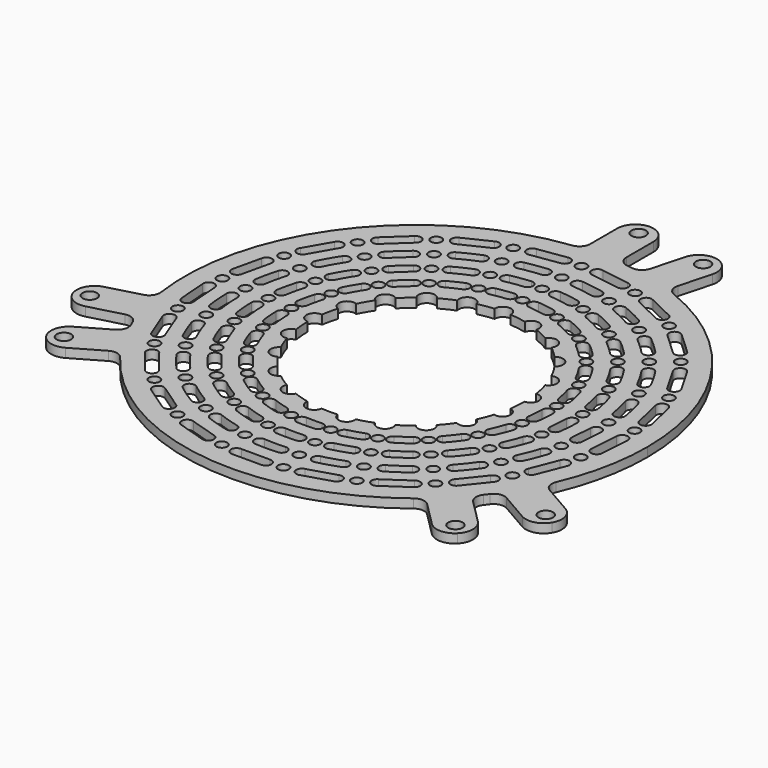
from build123d import *

# Parameters (mm, degrees)
F0_R      = 1.5
F0_R_2    = 30
F0_R_3    = 2
F1_DEPTH  = 2.5
F2_R      = 4.99999
F3_R      = 3
F5_DEPTH  = 25
F6_R      = 1.5579033755
F6_R_2    = 1.5577764336
F7_DEPTH  = 25
F8_R      = 2.25
F9_DEPTH  = 25
F11_DEPTH = 25
F12_R     = 1.5
F12_R_2   = 1.5000000369
F12_R_3   = 1.5000000493
F12_R_4   = 1.5000000692
F13_DEPTH = 25


# Not quite as in the source:
# - a fillet or chamfer is up to 0.001 mm smaller than in the source, because OpenCascade refuses the exact size


with BuildPart() as f1:
    # F0 (on Top) → F1 (new body)
    with BuildSketch(Plane.XY):
        with BuildLine():
            ThreePointArc((57.7562213692, -27.572067263), (62.4195408812, -14.1350951955), (64, 0))
            ThreePointArc((64, 0), (52.2588695026, 36.9460492923), (21.3434200529, 60.3362115188))
            ThreePointArc((21.3434200529, 60.3362115188), (16.5644188866, 61.8192528825), (11.68416179, 62.9244019699))
            ThreePointArc((11.68416179, 62.9244019699), (8.3536763021, 63.4524711279), (5, 63.8043885638))
            ThreePointArc((5, 63.8043885638), (0, 64), (-5, 63.8043885638))
            ThreePointArc((-5, 63.8043885638), (-50.7746137786, 38.9607314566), (-62.9244019699, -11.68416179))
            ThreePointArc((-62.9244019699, -11.68416179), (-61.8192528825, -16.5644188866), (-60.3362115188, -21.3434200529))
            ThreePointArc((-60.3362115188, -21.3434200529), (-59.1282900807, -24.4917396714), (-57.7562213692, -27.572067263))
            ThreePointArc((-57.7562213692, -27.572067263), (-55.4256258422, -32), (-52.7562213692, -36.2323213008))
            ThreePointArc((-52.7562213692, -36.2323213008), (-8.3536763021, -63.4524711279), (41.580981917, -48.6520497289))
            ThreePointArc((41.580981917, -48.6520497289), (45.2548339959, -45.2548339959), (48.6520497289, -41.580981917))
            ThreePointArc((48.6520497289, -41.580981917), (50.7746137786, -38.9607314566), (52.7562213692, -36.2323213008))
            ThreePointArc((52.7562213692, -36.2323213008), (55.4256258422, -32), (57.7562213692, -27.572067263))
        make_face()
        with Locations((-49.5366530965, -28.6)):
            Circle(F0_R, mode=Mode.SUBTRACT)
        with Locations((-24.8181498775, -51.535419244)):
            Circle(F0_R, mode=Mode.SUBTRACT)
        with Locations((-8.5252176253, -56.5611232601)):
            Circle(F0_R, mode=Mode.SUBTRACT)
        with Locations((-7.5117302153, -49.8370736417)):
            Circle(F0_R, mode=Mode.SUBTRACT)
        with Locations((-38.9058806005, -41.9305670687)):
            Circle(F0_R, mode=Mode.SUBTRACT)
        with Locations((-34.2807059837, -36.9458143402)):
            Circle(F0_R, mode=Mode.SUBTRACT)
        with Locations((-29.6555313668, -31.9610616118)):
            Circle(F0_R, mode=Mode.SUBTRACT)
        with Locations((-21.8677404515, -45.4088309423)):
            Circle(F0_R, mode=Mode.SUBTRACT)
        with Locations((-18.9173310255, -39.2822426405)):
            Circle(F0_R, mode=Mode.SUBTRACT)
        with Locations((-6.4982428053, -43.1130240234)):
            Circle(F0_R, mode=Mode.SUBTRACT)
        with Locations((-15.9669215995, -33.1556543388)):
            Circle(F0_R, mode=Mode.SUBTRACT)
        with Locations((-5.4847553953, -36.3889744051)):
            Circle(F0_R, mode=Mode.SUBTRACT)
        with Locations((-43.6476803507, -25.2)):
            Circle(F0_R, mode=Mode.SUBTRACT)
        with Locations((-55.7658765768, -12.7281974223)):
            Circle(F0_R, mode=Mode.SUBTRACT)
        with Locations((-49.136366774, -11.2150550714)):
            Circle(F0_R, mode=Mode.SUBTRACT)
        with Locations((-42.5068569711, -9.7019127205)):
            Circle(F0_R, mode=Mode.SUBTRACT)
        with Locations((-57.0400571988, 4.2745613531)):
            Circle(F0_R, mode=Mode.SUBTRACT)
        with Locations((-50.2590713779, 3.7663967168)):
            Circle(F0_R, mode=Mode.SUBTRACT)
        with Locations((-43.4780855571, 3.2582320804)):
            Circle(F0_R, mode=Mode.SUBTRACT)
        with Locations((-37.758707605, -21.8)):
            Circle(F0_R, mode=Mode.SUBTRACT)
        with Locations((-25.03035675, -26.9763088833)):
            Circle(F0_R, mode=Mode.SUBTRACT)
        with Locations((-31.8697348593, -18.4)):
            Circle(F0_R, mode=Mode.SUBTRACT)
        with Locations((-35.8773471683, -8.1887703696)):
            Circle(F0_R, mode=Mode.SUBTRACT)
        with Locations((-36.6970997363, 2.750067444)):
            Circle(F0_R, mode=Mode.SUBTRACT)
        with Locations((8.5252176253, -56.5611232601)):
            Circle(F0_R, mode=Mode.SUBTRACT)
        with Locations((7.5117302153, -49.8370736417)):
            Circle(F0_R, mode=Mode.SUBTRACT)
        with Locations((24.8181498775, -51.535419244)):
            Circle(F0_R, mode=Mode.SUBTRACT)
        with Locations((6.4982428053, -43.1130240234)):
            Circle(F0_R, mode=Mode.SUBTRACT)
        with Locations((5.4847553953, -36.3889744051)):
            Circle(F0_R, mode=Mode.SUBTRACT)
        with Locations((21.8677404515, -45.4088309423)):
            Circle(F0_R, mode=Mode.SUBTRACT)
        with Locations((18.9173310255, -39.2822426405)):
            Circle(F0_R, mode=Mode.SUBTRACT)
        with Locations((34.2807059837, -36.9458143402)):
            Circle(F0_R, mode=Mode.SUBTRACT)
        with Locations((15.9669215995, -33.1556543388)):
            Circle(F0_R, mode=Mode.SUBTRACT)
        with Locations((29.6555313668, -31.9610616118)):
            Circle(F0_R, mode=Mode.SUBTRACT)
        with Locations((38.9058806005, -41.9305670687)):
            Circle(F0_R, mode=Mode.SUBTRACT)
        with Locations((49.5366530965, -28.6)):
            Circle(F0_R, mode=Mode.SUBTRACT)
        with Locations((25.03035675, -26.9763088833)):
            Circle(F0_R, mode=Mode.SUBTRACT)
        with Locations((31.8697348593, -18.4)):
            Circle(F0_R, mode=Mode.SUBTRACT)
        Circle(F0_R_2, mode=Mode.SUBTRACT)
        with Locations((43.6476803507, -25.2)):
            Circle(F0_R, mode=Mode.SUBTRACT)
        with Locations((37.758707605, -21.8)):
            Circle(F0_R, mode=Mode.SUBTRACT)
        with Locations((42.5068569711, -9.7019127205)):
            Circle(F0_R, mode=Mode.SUBTRACT)
        with Locations((49.136366774, -11.2150550714)):
            Circle(F0_R, mode=Mode.SUBTRACT)
        with Locations((55.7658765768, -12.7281974223)):
            Circle(F0_R, mode=Mode.SUBTRACT)
        with Locations((35.8773471683, -8.1887703696)):
            Circle(F0_R, mode=Mode.SUBTRACT)
        with Locations((36.6970997363, 2.750067444)):
            Circle(F0_R, mode=Mode.SUBTRACT)
        with Locations((43.4780855571, 3.2582320804)):
            Circle(F0_R, mode=Mode.SUBTRACT)
        with Locations((50.2590713779, 3.7663967168)):
            Circle(F0_R, mode=Mode.SUBTRACT)
        with Locations((57.0400571988, 4.2745613531)):
            Circle(F0_R, mode=Mode.SUBTRACT)
        with Locations((-53.2459784224, 20.8975065938)):
            Circle(F0_R, mode=Mode.SUBTRACT)
        with Locations((-46.9160369317, 18.4131876281)):
            Circle(F0_R, mode=Mode.SUBTRACT)
        with Locations((-44.7207607972, 35.6636166663)):
            Circle(F0_R, mode=Mode.SUBTRACT)
        with Locations((-40.5860954409, 15.9288686624)):
            Circle(F0_R, mode=Mode.SUBTRACT)
        with Locations((-34.2561539501, 13.4445496967)):
            Circle(F0_R, mode=Mode.SUBTRACT)
        with Locations((-28.7713985548, 22.9444247084)):
            Circle(F0_R, mode=Mode.SUBTRACT)
        with Locations((-34.0878526356, 27.184155361)):
            Circle(F0_R, mode=Mode.SUBTRACT)
        with Locations((-39.4043067164, 31.4238860137)):
            Circle(F0_R, mode=Mode.SUBTRACT)
        with Locations((-24.5607545316, 36.0240105602)):
            Circle(F0_R, mode=Mode.SUBTRACT)
        with Locations((-28.3913309264, 41.6424342255)):
            Circle(F0_R, mode=Mode.SUBTRACT)
        with Locations((-20.7301781367, 30.4055868948)):
            Circle(F0_R, mode=Mode.SUBTRACT)
        with Locations((-10.8469904183, 35.1650792529)):
            Circle(F0_R, mode=Mode.SUBTRACT)
        with Locations((-12.8513256043, 41.6629743323)):
            Circle(F0_R, mode=Mode.SUBTRACT)
        with Locations((-32.2219073212, 47.2608578909)):
            Circle(F0_R, mode=Mode.SUBTRACT)
        with Locations((-14.8556607903, 48.1608694116)):
            Circle(F0_R, mode=Mode.SUBTRACT)
        with Locations((-16.8599959763, 54.658764491)):
            Circle(F0_R, mode=Mode.SUBTRACT)
        with Locations((34.2561539501, 13.4445496967)):
            Circle(F0_R, mode=Mode.SUBTRACT)
        with Locations((28.7713985548, 22.9444247084)):
            Circle(F0_R, mode=Mode.SUBTRACT)
        with Locations((10.8469904183, 35.1650792529)):
            Circle(F0_R, mode=Mode.SUBTRACT)
        with Locations((0, 36.8)):
            Circle(F0_R, mode=Mode.SUBTRACT)
        with Locations((0, 43.6)):
            Circle(F0_R, mode=Mode.SUBTRACT)
        with Locations((12.8513256043, 41.6629743323)):
            Circle(F0_R, mode=Mode.SUBTRACT)
        with Locations((20.7301781367, 30.4055868948)):
            Circle(F0_R, mode=Mode.SUBTRACT)
        with Locations((34.0878526356, 27.184155361)):
            Circle(F0_R, mode=Mode.SUBTRACT)
        with Locations((24.5607545316, 36.0240105602)):
            Circle(F0_R, mode=Mode.SUBTRACT)
        with Locations((28.3913309264, 41.6424342255)):
            Circle(F0_R, mode=Mode.SUBTRACT)
        with Locations((40.5860954409, 15.9288686624)):
            Circle(F0_R, mode=Mode.SUBTRACT)
        with Locations((46.9160369317, 18.4131876281)):
            Circle(F0_R, mode=Mode.SUBTRACT)
        with Locations((53.2459784224, 20.8975065938)):
            Circle(F0_R, mode=Mode.SUBTRACT)
        with Locations((39.4043067164, 31.4238860137)):
            Circle(F0_R, mode=Mode.SUBTRACT)
        with Locations((44.7207607972, 35.6636166663)):
            Circle(F0_R, mode=Mode.SUBTRACT)
        with Locations((0, 50.4)):
            Circle(F0_R, mode=Mode.SUBTRACT)
        with Locations((14.8556607903, 48.1608694116)):
            Circle(F0_R, mode=Mode.SUBTRACT)
        with Locations((0, 57.2)):
            Circle(F0_R, mode=Mode.SUBTRACT)
        with Locations((32.2219073212, 47.2608578909)):
            Circle(F0_R, mode=Mode.SUBTRACT)
        with Locations((16.8599959763, 54.658764491)):
            Circle(F0_R, mode=Mode.SUBTRACT)
        with BuildLine():
            ThreePointArc((-5, 63.8043885638), (0, 64), (5, 63.8043885638))
            Line((5, 63.8043885638), (5, 80.8455317256))
            Line((5, 80.8455317256), (-5, 80.8455317256))
            Line((-5, 80.8455317256), (-5, 63.8043885638))
        make_face()
        with Locations((0, 77)):
            Circle(F0_R_3, mode=Mode.SUBTRACT)
        with BuildLine():
            ThreePointArc((11.68416179, 62.9244019699), (16.5644188866, 61.8192528825), (21.3434200529, 60.3362115188))
            Line((21.3434200529, 60.3362115188), (25.7539924535, 76.7966918083))
            Line((25.7539924535, 76.7966918083), (16.0947341906, 79.3848822594))
            Line((16.0947341906, 79.3848822594), (11.68416179, 62.9244019699))
        make_face()
        with Locations((19.9290664729, 74.3762886243)):
            Circle(F0_R_3, mode=Mode.SUBTRACT)
        with BuildLine():
            Line((72.5142842569, -36.0926388439), (57.7562213692, -27.572067263))
            ThreePointArc((57.7562213692, -27.572067263), (55.4256258422, -32), (52.7562213692, -36.2323213008))
            Line((52.7562213692, -36.2323213008), (67.5142842569, -44.7528928817))
            Line((67.5142842569, -44.7528928817), (72.5142842569, -36.0926388439))
        make_face()
        with Locations((66.6839560914, -38.5)):
            Circle(F0_R_3, mode=Mode.SUBTRACT)
        with BuildLine():
            Line((60.7019576178, -53.6308898059), (48.6520497289, -41.580981917))
            ThreePointArc((48.6520497289, -41.580981917), (45.2548339959, -45.2548339959), (41.580981917, -48.6520497289))
            Line((41.580981917, -48.6520497289), (53.6308898059, -60.7019576178))
            Line((53.6308898059, -60.7019576178), (60.7019576178, -53.6308898059))
        make_face()
        with Locations((54.4472221514, -54.4472221514)):
            Circle(F0_R_3, mode=Mode.SUBTRACT)
        with BuildLine():
            Line((-67.5142842569, -44.7528928817), (-52.7562213692, -36.2323213008))
            ThreePointArc((-52.7562213692, -36.2323213008), (-55.4256258422, -32), (-57.7562213692, -27.572067263))
            Line((-57.7562213692, -27.572067263), (-72.5142842569, -36.0926388439))
            Line((-72.5142842569, -36.0926388439), (-67.5142842569, -44.7528928817))
        make_face()
        with Locations((-66.6839560914, -38.5)):
            Circle(F0_R_3, mode=Mode.SUBTRACT)
        with BuildLine():
            ThreePointArc((-60.3362115188, -21.3434200529), (-61.8192528825, -16.5644188866), (-62.9244019699, -11.68416179))
            Line((-62.9244019699, -11.68416179), (-79.3848822594, -16.0947341906))
            Line((-79.3848822594, -16.0947341906), (-76.7966918083, -25.7539924535))
            Line((-76.7966918083, -25.7539924535), (-60.3362115188, -21.3434200529))
        make_face()
        with Locations((-74.3762886243, -19.9290664729)):
            Circle(F0_R_3, mode=Mode.SUBTRACT)
    extrude(amount=F1_DEPTH)

    # F2 (radius 5 in the source; OpenCascade refuses exactly that, so slightly less here)
    f2_edges = [f1.edges().sort_by_distance(p)[0] for p in [
        (-5, 80.845532, 1.25),
        (5, 80.845532, 1.25),
        (16.094734, 79.384882, 1.25),
        (25.753992, 76.796692, 1.25),
        (-67.514284, -44.752893, 1.25),
        (-72.514284, -36.092639, 1.25),
        (-76.796692, -25.753992, 1.25),
        (-79.384882, -16.094734, 1.25),
        (60.701958, -53.63089, 1.25),
        (53.63089, -60.701958, 1.25),
        (67.514284, -44.752893, 1.25),
        (72.514284, -36.092639, 1.25),
    ]]
    fillet(f2_edges, radius=F2_R)

    # F3
    f3_edges = [f1.edges().sort_by_distance(p)[0] for p in [
        (5, 63.804389, 1.25),
        (-5, 63.804389, 1.25),
        (-57.756221, -27.572067, 1.25),
        (-62.924402, -11.684162, 1.25),
        (-52.756221, -36.232321, 1.25),
        (-60.336212, -21.34342, 1.25),
        (21.34342, 60.336212, 1.25),
        (11.684162, 62.924402, 1.25),
        (57.756221, -27.572067, 1.25),
        (48.65205, -41.580982, 1.25),
        (52.756221, -36.232321, 1.25),
        (41.580982, -48.65205, 1.25),
    ]]
    fillet(f3_edges, radius=F3_R)

    # F4 (on face) → F5 (cut)
    with BuildSketch(Plane.XY.offset(2.5)):
        Polygon((-36.8119077732, 45.824213326), (-42.9265368297, 40.1533001964), (-40.65668766, 38.01918342), (-34.8915175, 43.3705725804), align=None)
        Polygon((-48.6833819883, 32.9378718048), (-52.8548242436, 25.7165828801), (-50.0567761412, 24.3463287121), (-46.1250859609, 31.159284403), align=None)
        Polygon((-56.2291240703, 17.1248558283), (-58.0867285739, 8.9948343196), (-55.0091003916, 8.5101958561), (-53.2602381175, 16.1793570661), align=None)
        Polygon((-58.7786617212, -0.2097787398), (-58.1573721609, -8.5261447434), (-55.0736246688, -8.0821052481), (-55.6629843887, -0.238177148), align=None)
        Polygon((-56.1054573322, -17.5257735462), (-53.0604780121, -25.2895384295), (-50.2446157076, -23.9562758333), (-53.1198302239, -16.6345482773), align=None)
        Polygon((-48.4470368446, -33.2845264625), (-43.2489275398, -39.8058456449), (-40.9511521459, -37.7018261803), (-45.8567460312, -31.5528667926), align=None)
        Polygon((-36.4838845269, -46.0858031359), (-29.5945200608, -50.7852287897), (-28.0189990048, -48.0974038195), (-34.5190887147, -43.667574626), align=None)
        Polygon((-21.2789789622, -54.7921539564), (-13.310509601, -57.2521214892), (-12.5972348428, -54.2193160573), (-20.1142588813, -51.9022268218), align=None)
        Polygon((-4.1833427354, -58.6299814464), (4.1561980491, -58.6319119476), (3.943848917, -55.5236041259), (-3.9221888763, -55.5251383954), align=None)
        Polygon((13.2840018517, -57.2582777916), (21.2536092633, -54.8019997275), (20.1345043932, -51.8943763065), (12.6183848226, -54.2143977544), align=None)
        Polygon((29.5710045784, -50.7989248811), (36.4625440246, -46.102689337), (34.5361207953, -43.6541054177), (28.0377596551, -48.086469957), align=None)
        Polygon((43.2304937781, -39.8258645675), (48.431621736, -33.3069526807), (45.8690513055, -31.5349756895), (40.9658565006, -37.68584828), align=None)
        Polygon((53.0487638918, -25.3141014142), (56.0973373175, -17.5517471134), (53.1263153142, -16.6138249824), (50.2539572203, -23.9366736016), align=None)
        Polygon((58.1534185329, -8.5530692611), (58.7785582993, -0.2369917906), (55.6630730662, -0.2164630171), (55.0767733051, -8.0606204294), align=None)
        Polygon((58.0908867354, 8.9679406303), (56.2370464307, 17.0988212928), (53.2539225029, 16.2001326373), (55.0057763813, 8.5316542414), align=None)
        Polygon((52.8667247237, 25.6921096416), (48.6986261945, 32.9153290674), (46.1129272242, 31.1772754137), (50.0472748372, 24.3658539924), align=None)
        Polygon((42.9451222186, 40.1334219633), (36.8331193106, 45.8071654079), (34.8745959984, 43.3841804504), (40.6418532949, 38.0350406883), align=None)
        Polygon((29.2076571427, 51.0087036209), (21.6948281364, 54.6288340804), (20.5375038735, 51.7362106658), (27.6252247336, 48.324647105), align=None)
        Polygon((12.8749635541, 57.3516381138), (4.6288562761, 58.5964911102), (4.3755644021, 55.4912515228), (12.1539737234, 54.3203965573), align=None)
        Polygon((-4.6017270472, 58.5986278767), (-12.8484097777, 57.3575927584), (-12.1751631683, 54.3156511627), (-4.397211189, 55.4895403942), align=None)
        Polygon((-21.669534006, 54.638872397), (-29.1840382385, 51.0222205803), (-27.6440740613, 48.3138668365), (-20.5576845904, 51.7281950554), align=None)
    extrude(amount=-F5_DEPTH, mode=Mode.SUBTRACT)

    # F6 (on face) → F7 (cut)
    with BuildSketch(Plane.XY.offset(2.5)):
        with Locations((-57.2208230549, -0.2239779439)):
            Circle(F6_R)
        with Locations((-56.6154984149, -8.3041249957)):
            Circle(F6_R_2)
        with Locations((-54.6126437781, -17.0801609118)):
            Circle(F6_R)
        with Locations((-51.6525468599, -24.6229071314)):
            Circle(F6_R_2)
        with Locations((-47.1518914379, -32.4186966276)):
            Circle(F6_R)
        with Locations((-42.1000398428, -38.7538359126)):
            Circle(F6_R_2)
        with Locations((-35.5014866208, -44.8766888809)):
            Circle(F6_R)
        with Locations((-28.8067595328, -49.4413163046)):
            Circle(F6_R_2)
        with Locations((-20.6966189217, -53.3471903891)):
            Circle(F6_R)
        with Locations((-12.9538722219, -55.7357187732)):
            Circle(F6_R_2)
        with Locations((-4.0527658059, -57.0775599209)):
            Circle(F6_R)
        with Locations((4.050023483, -57.0777580367)):
            Circle(F6_R_2)
        with Locations((12.9511933371, -55.736337773)):
            Circle(F6_R)
        with Locations((20.6940568283, -53.348188017)):
            Circle(F6_R_2)
        with Locations((28.8043821168, -49.4426974191)):
            Circle(F6_R)
        with Locations((35.49933241, -44.8783973774)):
            Circle(F6_R_2)
        with Locations((42.0981751393, -38.7558564238)):
            Circle(F6_R)
        with Locations((47.1503365208, -32.4209641851)):
            Circle(F6_R_2)
        with Locations((51.651360556, -24.6253875079)):
            Circle(F6_R)
        with Locations((54.6118263158, -17.0827860479)):
            Circle(F6_R_2)
        with Locations((56.615095919, -8.3068448453)):
            Circle(F6_R)
        with Locations((57.2208156827, -0.2267274038)):
            Circle(F6_R_2)
        with Locations((56.5483315583, 8.7497974359)):
            Circle(F6_R)
        with Locations((54.7454844668, 16.6494769651)):
            Circle(F6_R_2)
        with Locations((51.4569997805, 25.028981817)):
            Circle(F6_R)
        with Locations((47.4057767094, 32.0463022406)):
            Circle(F6_R_2)
        with Locations((41.7934877568, 39.0842313258)):
            Circle(F6_R)
        with Locations((35.8538576545, 44.5956729292)):
            Circle(F6_R_2)
        with Locations((28.4164409382, 49.666675363)):
            Circle(F6_R)
        with Locations((21.1161660049, 53.1825223731)):
            Circle(F6_R_2)
        with Locations((12.5144686387, 55.8360173355)):
            Circle(F6_R)
        with Locations((4.5022103391, 57.0438713165)):
            Circle(F6_R_2)
        with Locations((-4.4994691181, 57.0440841355)):
            Circle(F6_R)
        with Locations((-12.511786473, 55.8366219606)):
            Circle(F6_R_2)
        with Locations((-21.1136092982, 53.1835337262)):
            Circle(F6_R)
        with Locations((-28.4140561499, 49.6680437084)):
            Circle(F6_R_2)
        with Locations((-35.8517126366, 44.5973929532)):
            Circle(F6_R)
        with Locations((-41.7916122449, 39.0862418082)):
            Circle(F6_R_2)
        with Locations((-47.4042339746, 32.0485781039)):
            Circle(F6_R)
        with Locations((-51.4558001924, 25.0314557961)):
            Circle(F6_R_2)
        with Locations((-54.7446810939, 16.6521064472)):
            Circle(F6_R)
        with Locations((-56.5479144828, 8.7525150879)):
            Circle(F6_R_2)
    extrude(amount=-F7_DEPTH, mode=Mode.SUBTRACT)

    # F8 (on face) → F9 (cut)
    with BuildSketch(Plane.XY.offset(2.5)):
        with Locations((16.8996017419, 24.7871632295)):
            Circle(F8_R)
        with Locations((8.8426552323, 28.6671841736)):
            Circle(F8_R)
        with Locations((0, 30)):
            Circle(F8_R)
        with Locations((-8.8426552323, 28.6671841736)):
            Circle(F8_R)
        with Locations((-16.8996017419, 24.7871632295)):
            Circle(F8_R)
        with Locations((-23.454944474, 18.7046940558)):
            Circle(F8_R)
        with Locations((-27.9262124593, 10.960230731)):
            Circle(F8_R)
        with Locations((-29.9161139154, 2.2419028076)):
            Circle(F8_R)
        with Locations((-29.2478373655, -6.6756280187)):
            Circle(F8_R)
        with Locations((-25.9807621135, -15)):
            Circle(F8_R)
        with Locations((-20.4051821331, -21.9915561549)):
            Circle(F8_R)
        with Locations((-13.0165121735, -27.0290660371)):
            Circle(F8_R)
        with Locations((-4.4712679853, -29.6649247868)):
            Circle(F8_R)
        with Locations((4.4712679853, -29.6649247868)):
            Circle(F8_R)
        with Locations((13.0165121735, -27.0290660371)):
            Circle(F8_R)
        with Locations((20.4051821331, -21.9915561549)):
            Circle(F8_R)
        with Locations((25.9807621135, -15)):
            Circle(F8_R)
        with Locations((29.2478373655, -6.6756280187)):
            Circle(F8_R)
        with Locations((29.9161139154, 2.2419028076)):
            Circle(F8_R)
        with Locations((27.9262124593, 10.960230731)):
            Circle(F8_R)
        with Locations((23.454944474, 18.7046940558)):
            Circle(F8_R)
    extrude(amount=-F9_DEPTH, mode=Mode.SUBTRACT)

    # F10 (on face) → F11 (cut)
    with BuildSketch(Plane.XY.offset(2.5)):
        with BuildLine():
            Line((41.7169760554, -5.6660311324), (44.6896821876, -6.06978632))
            ThreePointArc((44.6896821876, -6.06978632), (44.97384885, -3.3708929995), (45.0951734833, -0.6597942959))
            Line((45.0951734833, -0.6597942959), (42.0954836602, -0.6166485343))
            Line((42.0954836602, -0.6166485343), (41.7169760554, -5.6660311324))
        make_face()
        with BuildLine():
            Line((34.9788421557, -4.7508527072), (37.9515482879, -5.1546078948))
            ThreePointArc((37.9515482879, -5.1546078948), (38.1928064688, -2.8634828512), (38.2958765288, -0.5619972359))
            Line((38.2958765288, -0.5619972359), (35.2961866658, -0.5188514737))
            ThreePointArc((35.2961866658, -0.5188514737), (35.2011701166, -2.6396254323), (34.9788421557, -4.7508527072))
        make_face()
        Polygon((51.8944703734, -0.7575913551), (48.8947805752, -0.7144455938), (48.4551099551, -6.5812095576), (51.4278160873, -6.9849647451), align=None)
        with BuildLine():
            Line((49.8122486315, 14.5722299691), (46.9331091981, 13.7292847956))
            ThreePointArc((46.9331091981, 13.7292847956), (47.6740070724, 10.881132738), (48.2422309454, 7.9935695035))
            Line((48.2422309454, 7.9935695035), (51.2018770157, 8.4839725405))
            ThreePointArc((51.2018770157, 8.4839725405), (50.5987165321, 11.5490209673), (49.8122486315, 14.5722299691))
        make_face()
        with BuildLine():
            Line((34.8251687602, 5.770409069), (37.7848148305, 6.260812106))
            ThreePointArc((37.7848148305, 6.260812106), (37.3400336254, 8.5212609895), (36.7601497779, 10.7508784899))
            Line((36.7601497779, 10.7508784899), (33.8810102824, 9.9079332983))
            ThreePointArc((33.8810102824, 9.9079332983), (34.4153241499, 7.8533727566), (34.8251687602, 5.770409069))
        make_face()
        with BuildLine():
            Line((43.2861992356, 12.6615542385), (40.4070597784, 11.8186090581))
            ThreePointArc((40.4070597784, 11.8186090581), (41.0446656208, 9.3672527495), (41.5336998528, 6.8819892863))
            Line((41.5336998528, 6.8819892863), (44.4933459231, 7.3723923233))
            ThreePointArc((44.4933459231, 7.3723923233), (43.9693750866, 10.0351409802), (43.2861992356, 12.6615542385))
        make_face()
        with BuildLine():
            Line((43.3039900013, 28.6072447113), (40.8012251063, 26.9531079809))
            ThreePointArc((40.8012251063, 26.9531079809), (42.3487145232, 24.4498748101), (43.7428180087, 21.858084835))
            Line((43.7428180087, 21.858084835), (46.4264264755, 23.1990716347))
            ThreePointArc((46.4264264755, 23.1990716347), (44.9466238363, 25.9501638862), (43.3039900013, 28.6072447113))
        make_face()
        with BuildLine():
            Line((31.5771262926, 15.7789446764), (34.2607347594, 17.1199314761))
            ThreePointArc((34.2607347594, 17.1199314761), (33.1694349305, 19.1488533963), (31.9581224, 21.1084914824))
            Line((31.9581224, 21.1084914824), (29.4553574511, 19.4543547164))
            ThreePointArc((29.4553574511, 19.4543547164), (30.5715256034, 17.6485643121), (31.5771262926, 15.7789446764))
        make_face()
        with BuildLine():
            Line((37.6310562275, 24.8578681146), (35.1282913118, 23.2037313705))
            ThreePointArc((35.1282913118, 23.2037313705), (36.4601200719, 21.0492195661), (37.6599721507, 18.8185147557))
            Line((37.6599721507, 18.8185147557), (40.3435806175, 20.1595015554))
            ThreePointArc((40.3435806175, 20.1595015554), (39.0580293903, 22.5495086453), (37.6310562275, 24.8578681146))
        make_face()
        with BuildLine():
            Line((25.52331758, 24.3854518045), (27.6924380542, 26.4578698049))
            ThreePointArc((27.6924380542, 26.4578698049), (26.0515863802, 28.0749861455), (24.316475601, 29.5905223737))
            Line((24.316475601, 29.5905223737), (22.4124668475, 27.2721713439))
            ThreePointArc((22.4124668475, 27.2721713439), (24.0113128461, 25.8756034791), (25.52331758, 24.3854518045))
        make_face()
        with BuildLine():
            Line((32.9479818229, 40.1003802201), (31.0439731105, 37.7820292403))
            ThreePointArc((31.0439731105, 37.7820292403), (33.2605528444, 35.8461382088), (35.3566637298, 33.7804134063))
            Line((35.3566637298, 33.7804134063), (37.525784204, 35.8528314067))
            ThreePointArc((37.525784204, 35.8528314067), (35.3008263676, 38.0455208634), (32.9479818229, 40.1003802201))
        make_face()
        with BuildLine():
            Line((28.6322287324, 34.8454513217), (26.7282200042, 32.5271003228))
            ThreePointArc((26.7282200042, 32.5271003228), (28.635932852, 30.8608708512), (30.4399906549, 29.0829326054))
            Line((30.4399906549, 29.0829326054), (32.6091111291, 31.1553506058))
            ThreePointArc((32.6091111291, 31.1553506058), (30.6762063794, 33.0602535104), (28.6322287324, 34.8454513217))
        make_face()
        with BuildLine():
            Line((17.2016500931, 30.8252045261), (18.6635467016, 33.4449102932))
            ThreePointArc((18.6635467016, 33.4449102931), (16.6189400546, 34.5065331707), (14.5142032337, 35.4433054961))
            Line((14.5142032337, 35.4433054961), (13.378130209, 32.6667358656))
            ThreePointArc((13.378130209, 32.6667358656), (15.3175895705, 31.8034817237), (17.2016500931, 30.8252045261))
        make_face()
        with BuildLine():
            Line((19.6644008698, 48.0304209687), (18.5283278696, 45.253851398))
            ThreePointArc((18.5283278696, 45.253851398), (21.2170450839, 44.0573149194), (23.8289147182, 42.7012040035))
            Line((23.8289147182, 42.7012040035), (25.2908113267, 45.3209097706))
            ThreePointArc((25.2908113267, 45.3209097706), (22.518395561, 46.7603663518), (19.6644008698, 48.0304209687))
        make_face()
        with BuildLine():
            Line((17.089302064, 41.7368632622), (15.9532290543, 38.9602936686))
            ThreePointArc((15.9532290543, 38.9602936686), (18.2673173315, 37.9303983305), (20.5152824057, 36.7632042648))
            Line((20.5152824057, 36.7632042648), (21.9771790142, 39.3829100319))
            ThreePointArc((21.9771790142, 39.3829100319), (19.5686678113, 40.6334497685), (17.089302064, 41.7368632622))
        make_face()
        with BuildLine():
            Line((7.3515405073, 34.5260025513), (7.976317321, 37.4602237313))
            ThreePointArc((7.976317321, 37.4602237312), (5.7096279742, 37.8720232942), (3.4222802146, 38.1467953848))
            Line((3.4222802146, 38.1467953848), (3.1550879925, 35.15871755))
            ThreePointArc((3.1550879925, 35.15871755), (5.2628312414, 34.9054810499), (7.3515405073, 34.5260025513))
        make_face()
        with BuildLine():
            Line((4.6335516036, 51.6927480362), (4.3663593873, 48.7046702658))
            ThreePointArc((4.3663593873, 48.7046702658), (7.2883097581, 48.3538058571), (10.1838620625, 47.8278052339))
            Line((10.1838620625, 47.8278052339), (10.8086388762, 50.7620264139))
            ThreePointArc((10.8086388762, 50.7620264139), (7.7351064885, 51.3203480854), (4.6335516036, 51.6927480362))
        make_face()
        with BuildLine():
            Line((4.027915912, 44.9197717426), (3.7607236934, 41.9316939474))
            ThreePointArc((3.7607236934, 41.9316939474), (6.2755705013, 41.6296434633), (8.7677012849, 41.1769038926))
            Line((8.7677012849, 41.1769038926), (9.3924780986, 44.1111250726))
            ThreePointArc((9.3924780986, 44.1111250726), (6.7223672325, 44.5961856978), (4.027915912, 44.9197717426))
        make_face()
        with BuildLine():
            Line((-3.1517857143, 35.1590137349), (-3.4196428571, 38.1470318993))
            ThreePointArc((-3.4196428571, 38.1470318993), (-5.7070096081, 37.8724179494), (-7.97372742, 37.4607750992))
            Line((-7.97372742, 37.4607750992), (-7.348297638, 34.5266928886))
            ThreePointArc((-7.348297638, 34.5266928886), (-5.259552739, 34.9059752046), (-3.1517857143, 35.1590137349))
        make_face()
        with BuildLine():
            Line((-10.8090090566, 50.7619475908), (-10.1835792881, 47.8278654435))
            ThreePointArc((-10.1835792881, 47.8278654435), (-7.2880238738, 48.3538489473), (-4.3660714286, 48.7046960804))
            Line((-4.3660714286, 48.7046960804), (-4.6339285714, 51.6927142448))
            ThreePointArc((-4.6339285714, 51.6927142448), (-7.7354807405, 51.320291676), (-10.8090090566, 50.7619475908))
        make_face()
        with BuildLine():
            Line((-9.391368245, 44.1113613765), (-8.7659384713, 41.1772792049))
            ThreePointArc((-8.7659384713, 41.1772792049), (-6.2737883079, 41.6299120858), (-3.7589285714, 41.9318549076))
            Line((-3.7589285714, 41.9318549076), (-4.0267857143, 44.9198730721))
            ThreePointArc((-4.0267857143, 44.9198730721), (-6.7212451755, 44.5963548207), (-9.391368245, 44.1113613765))
        make_face()
        with BuildLine():
            Line((-13.3750619438, 32.6679922554), (-14.5117527605, 35.4443088777))
            ThreePointArc((-14.5117527605, 35.4443088777), (-16.6165543419, 34.5076820694), (-18.6612343813, 33.446200552))
            Line((-18.6612343813, 33.446200552), (-17.1987547759, 30.8268200461))
            ThreePointArc((-17.1987547759, 30.8268200461), (-15.3146023774, 31.8049202801), (-13.3750619438, 32.6679922554))
        make_face()
        with BuildLine():
            Line((-25.2911418275, 45.3207253369), (-23.8286622537, 42.7013448875))
            ThreePointArc((-23.8286622537, 42.7013448875), (-21.2167846016, 44.0574403611), (-18.5280603131, 45.2539609431))
            Line((-18.5280603131, 45.2539609431), (-19.6647511298, 48.0302775653))
            ThreePointArc((-19.6647511298, 48.0302775653), (-22.5187365591, 46.7602021358), (-25.2911418275, 45.3207253369))
        make_face()
        with BuildLine():
            Line((-21.9761881201, 39.3834629726), (-20.5137085342, 36.7640825015))
            ThreePointArc((-20.5137085342, 36.7640825015), (-18.2656934938, 37.9311803295), (-15.9515611284, 38.9609765992))
            Line((-15.9515611284, 38.9609765992), (-17.0882519452, 41.7372932215))
            ThreePointArc((-17.0882519452, 41.7372932215), (-19.567645454, 40.6339421099), (-21.9761881201, 39.3834629726))
        make_face()
        with BuildLine():
            Line((-22.4099052241, 27.2742763029), (-24.3144297474, 29.5922034675))
            ThreePointArc((-24.3144297474, 29.5922034675), (-26.0496453019, 28.0767872031), (-27.6906087742, 26.4597843096))
            Line((-27.6906087742, 26.4597843096), (-25.5210270765, 24.3878489613))
            ThreePointArc((-25.5210270765, 24.3878489613), (-24.0088823876, 25.877858615), (-22.4099052241, 27.2742763029))
        make_face()
        with BuildLine():
            Line((-37.5260456588, 35.85255775), (-35.3564640078, 33.7806224464))
            ThreePointArc((-35.3564640078, 33.7806224464), (-33.2603409093, 35.8463348559), (-31.0437497297, 37.7822127822))
            Line((-31.0437497297, 37.7822127822), (-32.948274253, 40.1001399468))
            ThreePointArc((-32.948274253, 40.1001399468), (-35.3011038126, 38.0452634321), (-37.5260456588, 35.85255775))
        make_face()
        with BuildLine():
            Line((-32.6083272398, 31.156171052), (-30.4387455709, 29.0842357313))
            ThreePointArc((-30.4387455709, 29.0842357313), (-28.6346116552, 30.8620967427), (-26.7268274769, 32.5282445426))
            Line((-26.7268274769, 32.5282445426), (-28.6313520002, 34.8461717071))
            ThreePointArc((-28.6313520002, 34.8461717071), (-30.6753745627, 33.0610253235), (-32.6083272398, 31.156171052))
        make_face()
        with BuildLine():
            Line((-29.453530081, 19.4571212097), (-31.956662949, 21.1107009159))
            ThreePointArc((-31.956662949, 21.1107009159), (-33.1681109598, 19.1511465808), (-34.2595510594, 17.1223001145))
            Line((-34.2595510594, 17.1223001145), (-31.5756441241, 15.781910472))
            ThreePointArc((-31.5756441241, 15.781910472), (-30.5698678363, 17.6514356489), (-29.453530081, 19.4571212097))
        make_face()
        with BuildLine():
            Line((-46.4265956529, 23.1987330707), (-43.7426887755, 21.8583434571))
            ThreePointArc((-43.7426887755, 21.8583434571), (-42.3485699665, 24.4501251897), (-40.8010657496, 26.9533492112))
            Line((-40.8010657496, 26.9533492112), (-43.3041986176, 28.6069289174))
            ThreePointArc((-43.3041986176, 28.6069289174), (-44.9468130759, 25.9498361135), (-46.4265956529, 23.1987330707))
        make_face()
        with BuildLine():
            Line((-40.3430733849, 20.1605166069), (-37.6591664853, 18.8201269823))
            ThreePointArc((-37.6591664853, 18.8201269823), (-36.45921891, 21.0507804243), (-35.1272979153, 23.2052352104))
            Line((-35.1272979153, 23.2052352104), (-37.6304307833, 24.8588149166))
            ThreePointArc((-37.6304307833, 24.8588149166), (-39.0574620248, 22.5504913512), (-40.3430733849, 20.1605166069))
        make_face()
        with BuildLine():
            Line((-33.8800795355, 9.9111155108), (-36.7594064082, 10.7534199452))
            ThreePointArc((-36.7594064082, 10.7534199452), (-37.3394444031, 8.5238425414), (-37.7843818873, 6.2634244141))
            Line((-37.7843818873, 6.2634244141), (-34.8246266239, 5.7736799794))
            ThreePointArc((-34.8246266239, 5.7736799794), (-34.4145863742, 7.8566051634), (-33.8800795355, 9.9111155108))
        make_face()
        with BuildLine():
            Line((-51.2019388835, 8.4835991521), (-48.2421836839, 7.9938547279))
            ThreePointArc((-48.2421836839, 7.9938547279), (-47.6739427386, 10.8814146028), (-46.9330280251, 13.7295622799))
            Line((-46.9330280251, 13.7295622799), (-49.8123548978, 14.5718667142))
            ThreePointArc((-49.8123548978, 14.5718667142), (-50.5988007517, 11.5486519772), (-51.2019388835, 8.4835991521))
        make_face()
        with BuildLine():
            Line((-44.4931604172, 7.3735117884), (-41.5334051931, 6.8837673602))
            ThreePointArc((-41.5334051931, 6.8837673602), (-41.0442645661, 9.3690098853), (-40.4065537803, 11.8203388954))
            Line((-40.4065537803, 11.8203388954), (-43.285880653, 12.6626433297))
            ThreePointArc((-43.285880653, 12.6626433297), (-43.9691225852, 10.0362472611), (-44.4931604172, 7.3735117884))
        make_face()
        with BuildLine():
            Line((-35.296235243, -0.5155362954), (-38.295915292, -0.5593495783))
            ThreePointArc((-38.295915292, -0.5593495783), (-38.1930043497, -2.8608423141), (-37.9519045706, -5.151984032))
            Line((-37.9519045706, -5.151984032), (-34.9792882228, -4.7475673167))
            ThreePointArc((-34.9792882228, -4.7475673167), (-35.2014178868, -2.6363191691), (-35.296235243, -0.5155362954))
        make_face()
        with BuildLine():
            Line((-51.4277651483, -6.9853397809), (-48.4551488646, -6.5809230743))
            ThreePointArc((-48.4551488646, -6.5809230743), (-48.7632764847, -3.6541574238), (-48.8947847984, -0.7141565112))
            Line((-48.8947847984, -0.7141565112), (-51.8944648473, -0.757969794))
            ThreePointArc((-51.8944648473, -0.757969794), (-51.7548629315, -3.8786805676), (-51.4277651483, -6.9853397809))
        make_face()
        with BuildLine():
            Line((-44.6898348913, -6.0686619108), (-41.717218583, -5.6642452008))
            ThreePointArc((-41.717218583, -5.6642452008), (-41.9823471956, -3.1452382972), (-42.0955100207, -0.6148464033))
            Line((-42.0955100207, -0.6148464033), (-45.0951900696, -0.6586596862))
            ThreePointArc((-45.0951900696, -0.6586596862), (-44.9739336486, -3.3697614414), (-44.6898348913, -6.0686619108))
        make_face()
        with BuildLine():
            Line((-33.5761655542, -10.8963804393), (-36.4296640432, -11.822418437))
            ThreePointArc((-36.4296640432, -11.822418437), (-35.6529482526, -13.9913287753), (-34.7472339835, -16.1096160877))
            Line((-34.7472339835, -16.1096160877), (-32.025886559, -14.8469724223))
            ThreePointArc((-32.025886559, -14.8469724223), (-32.8604489412, -12.8949949741), (-33.5761655542, -10.8963804393))
        make_face()
        with BuildLine():
            Line((-47.0840087926, -21.8336006196), (-44.3626614268, -20.5709569815))
            ThreePointArc((-44.3626614268, -20.5709569815), (-45.519779121, -17.8650415274), (-46.5120253711, -15.0944193622))
            Line((-46.5120253711, -15.0944193622), (-49.3655238601, -16.0204573598))
            ThreePointArc((-49.3655238601, -16.0204573598), (-48.3122784173, -18.9613753227), (-47.0840087926, -21.8336006196))
        make_face()
        with BuildLine():
            Line((-40.9156214173, -18.9716083672), (-38.1942740289, -17.7089647186))
            ThreePointArc((-38.1942740289, -17.7089647186), (-39.1901140404, -15.3800182543), (-40.0440954626, -12.9953999008))
            Line((-40.0440954626, -12.9953999008), (-42.8975939516, -13.9214378984))
            ThreePointArc((-42.8975939516, -13.9214378984), (-41.9826133424, -16.476352052), (-40.9156214173, -18.9716083672))
        make_face()
        with BuildLine():
            Line((-28.8727062093, -20.3090333633), (-31.3264772752, -22.0350135358))
            ThreePointArc((-31.3264772752, -22.0350135358), (-29.9449712429, -23.878624275), (-28.4551191713, -25.6358380582))
            Line((-28.4551191713, -25.6358380582), (-26.2268443312, -23.6271588734))
            ThreePointArc((-26.2268443312, -23.6271588734), (-27.5996849016, -22.0078938868), (-28.8727062093, -20.3090333633))
        make_face()
        with BuildLine():
            Line((-38.556631631, -34.7418502281), (-36.3283568389, -32.7331710867))
            ThreePointArc((-36.3283568389, -32.7331710867), (-38.2316496222, -30.4885382917), (-39.9964683749, -28.1334768121))
            Line((-39.9964683749, -28.1334768121), (-42.4502394409, -29.8594569846))
            ThreePointArc((-42.4502394409, -29.8594569846), (-40.5769359508, -32.3592686698), (-38.556631631, -34.7418502281))
        make_face()
        with BuildLine():
            Line((-33.505875425, -30.1888441647), (-31.2776006145, -28.1801650066))
            ThreePointArc((-31.2776006145, -28.1801650066), (-32.9156672696, -26.2482160955), (-34.4345872921, -24.2212550877))
            Line((-34.4345872921, -24.2212550877), (-36.888358358, -25.9472352602))
            ThreePointArc((-36.888358358, -25.9472352602), (-35.2609536031, -28.1189464774), (-33.505875425, -30.1888441647))
        make_face()
        with BuildLine():
            Line((-21.6037802119, -27.9171395482), (-23.4397955274, -30.2897009829))
            ThreePointArc((-23.4397955274, -30.2897009829), (-21.5762521269, -31.6441992182), (-19.6346421475, -32.8842033162))
            Line((-19.6346421475, -32.8842033162), (-18.0974318899, -30.3079685725))
            ThreePointArc((-18.0974318899, -30.3079685725), (-19.8865677392, -29.1652948477), (-21.6037802119, -27.9171395482))
        make_face()
        with BuildLine():
            Line((-26.6033285459, -44.5631339818), (-25.0661183214, -41.9868992937))
            ThreePointArc((-25.0661183214, -41.9868992937), (-27.5464702776, -40.4029946322), (-29.927049642, -38.6727513855))
            Line((-29.927049642, -38.6727513855), (-31.7630649575, -41.0453128202))
            ThreePointArc((-31.7630649575, -41.0453128202), (-29.2361546562, -42.8818989892), (-26.6033285459, -44.5631339818))
        make_face()
        with BuildLine():
            Line((-23.1189853632, -38.7236686766), (-21.581775126, -36.1474339672))
            ThreePointArc((-21.581775126, -36.1474339672), (-23.716519014, -34.7841447482), (-25.765414927, -33.2949454669))
            Line((-25.765414927, -33.2949454669), (-27.6014302424, -35.6675069015))
            ThreePointArc((-27.6014302424, -35.6675069015), (-25.406203396, -37.2630491103), (-23.1189853632, -38.7236686766))
        make_face()
        with BuildLine():
            Line((-12.4152635361, -33.0446853719), (-13.4703850831, -35.8530155735))
            ThreePointArc((-13.4703850831, -35.8530155735), (-11.2903883236, -36.5980481925), (-9.0695410037, -37.2106627996))
            Line((-9.0695410037, -37.2106627996), (-8.3599832059, -34.2957822596))
            ThreePointArc((-8.3599832059, -34.2957822596), (-10.4064417624, -33.7312313716), (-12.4152635361, -33.0446853719))
        make_face()
        with BuildLine():
            Line((-12.2862029728, -50.4247877191), (-11.5766451903, -47.5099072419))
            ThreePointArc((-11.5766451903, -47.5099072419), (-14.4136661631, -46.7274675939), (-17.1984812158, -45.7757822857))
            Line((-17.1984812158, -45.7757822857), (-18.2536027627, -48.5841124873))
            ThreePointArc((-18.2536027627, -48.5841124873), (-15.2976127196, -49.5942843993), (-12.2862029728, -50.4247877191))
        make_face()
        with BuildLine():
            Line((-10.6778719958, -43.8177252906), (-9.9683142075, -40.9028447893))
            ThreePointArc((-9.9683142075, -40.9028447893), (-12.4100539657, -40.2293494922), (-14.8068723759, -39.4102338288))
            Line((-14.8068723759, -39.4102338288), (-15.8619939229, -42.2185640304))
            ThreePointArc((-15.8619939229, -42.2185640304), (-13.2940005239, -43.0961663036), (-10.6778719958, -43.8177252906))
        make_face()
        with BuildLine():
            Line((-2.1235962116, -35.2360658861), (-2.3040718103, -38.230632392))
            ThreePointArc((-2.3040718103, -38.230632392), (-0.0013239707, -38.2999999771), (2.3014286593, -38.2307915969))
            Line((2.3014286593, -38.2307915969), (2.1202866731, -35.2362651884))
            ThreePointArc((2.1202866731, -35.2362651884), (-0.0016577671, -35.2999999611), (-2.1235962116, -35.2360658861))
        make_face()
        with BuildLine():
            Line((3.1226056516, -51.805977782), (2.9414636693, -48.811451438))
            ThreePointArc((2.9414636693, -48.811451438), (-0.0001445567, -48.8999999998), (-2.9417522592, -48.8114340462))
            Line((-2.9417522592, -48.8114340462), (-3.1222278579, -51.8060005521))
            ThreePointArc((-3.1222278579, -51.8060005521), (0.0001892397, -51.8999999997), (3.1226056516, -51.805977782))
        make_face()
        with BuildLine():
            Line((2.7120171574, -45.0183847216), (2.5308751736, -42.0238583528))
            ThreePointArc((2.5308751736, -42.0238583528), (-0.0009011619, -42.0999999904), (-2.5326742354, -42.0237499661))
            Line((-2.5326742354, -42.0237499661), (-2.7131498341, -45.018316472))
            ThreePointArc((-2.7131498341, -45.018316472), (-0.0005673655, -45.0999999964), (2.7120171574, -45.0183847216))
        make_face()
        with BuildLine():
            Line((8.3567619555, -34.2965673154), (9.066968354, -37.2112897501))
            ThreePointArc((9.066968354, -37.2112897501), (11.2878580228, -36.598828687), (13.4679062863, -35.8539467878))
            Line((13.4679062863, -35.8539467878), (12.4121597764, -33.0458513233))
            ThreePointArc((12.4121597764, -33.0458513233), (10.4032735281, -33.7322086425), (8.3567619555, -34.2965673154))
        make_face()
        with BuildLine():
            Line((18.2539570605, -48.5839793721), (17.1982105734, -45.7758839682))
            ThreePointArc((17.1982105734, -45.7758839682), (14.4133898941, -46.7275528116), (11.5763642953, -47.5099756862))
            Line((11.5763642953, -47.5099756862), (12.2865706938, -50.4246981209))
            ThreePointArc((12.2865706938, -50.4246981209), (15.2979743841, -49.5941728406), (18.2539570605, -48.5839793721))
        make_face()
        with BuildLine():
            Line((15.8609316848, -42.2189631101), (14.8051851889, -39.4108676829))
            ThreePointArc((14.8051851889, -39.4108676829), (12.408331714, -40.2298807365), (9.9665631254, -40.9032715008))
            Line((9.9665631254, -40.9032715008), (10.6767695239, -43.8179939355))
            ThreePointArc((10.6767695239, -43.8179939355), (13.2929162058, -43.0965007715), (15.8609316848, -42.2189631101))
        make_face()
        with BuildLine():
            Line((18.0945851499, -30.3096682307), (19.6323685904, -32.8855607149))
            ThreePointArc((19.6323685904, -32.8855607149), (21.574064295, -31.6456908566), (23.4377013369, -30.2913214641))
            Line((23.4377013369, -30.2913214641), (21.6011580138, -27.9191685489))
            ThreePointArc((21.6011580138, -27.9191685489), (19.8838283163, -29.1671625546), (18.0945851499, -30.3096682307))
        make_face()
        with BuildLine():
            Line((31.7633642784, -41.0450811878), (29.926820995, -38.6729283237))
            ThreePointArc((29.926820995, -38.6729283237), (27.5462314008, -40.4031574956), (25.0658700801, -41.9870474924))
            Line((25.0658700801, -41.9870474924), (26.6036535206, -44.5629399766))
            ThreePointArc((26.6036535206, -44.5629399766), (29.2364673704, -42.8816857842), (31.7633642784, -41.0450811878))
        make_face()
        with BuildLine():
            Line((27.6005328274, -35.6682013514), (25.7639895287, -33.2960484677))
            ThreePointArc((25.7639895287, -33.2960484677), (23.7150298641, -34.7851600333), (21.580227615, -36.1483578615))
            Line((21.580227615, -36.1483578615), (23.1180110555, -38.7242503457))
            ThreePointArc((23.1180110555, -38.7242503457), (25.4052658373, -37.2636883271), (27.6005328274, -35.6682013514))
        make_face()
        with BuildLine():
            Line((26.2246250469, -23.6296221119), (28.4533467222, -25.6378052942))
            ThreePointArc((28.4533467222, -25.6378052942), (29.9433202784, -23.8806945189), (31.3249537689, -22.0371792971))
            Line((31.3249537689, -22.0371792971), (28.8707985665, -20.3117451277))
            ThreePointArc((28.8707985665, -20.3117451277), (27.5976176998, -22.0104860758), (26.2246250469, -23.6296221119))
        make_face()
        with BuildLine():
            Line((42.450457189, -29.8591474166), (39.9963020395, -28.1337132843))
            ThreePointArc((39.9963020395, -28.1337132843), (38.2314693629, -30.4887643298), (36.3281633085, -32.7333858717))
            Line((36.3281633085, -32.7333858717), (38.5568849839, -34.7415690541))
            ThreePointArc((38.5568849839, -34.7415690541), (40.5771719288, -32.3589727627), (42.450457189, -29.8591474166))
        make_face()
        with BuildLine():
            Line((36.8877055053, -25.9481633754), (34.4335503355, -24.2227292288))
            ThreePointArc((34.4335503355, -24.2227292288), (32.9145435391, -26.249625209), (31.2763941777, -28.1815039918))
            Line((31.2763941777, -28.1815039918), (33.5051158531, -30.1896871741))
            ThreePointArc((33.5051158531, -30.1896871741), (35.2602461099, -28.1198336458), (36.8877055053, -25.9481633754))
        make_face()
        with BuildLine():
            Line((32.0244919236, -14.8499803716), (34.7461201324, -16.1120183635))
            ThreePointArc((34.7461201324, -16.1120183635), (35.651980851, -13.9937936744), (36.4288465914, -11.824937041))
            Line((36.4288465914, -11.824937041), (33.5751419692, -10.8995340152))
            ThreePointArc((33.5751419692, -10.8995340152), (32.8592376406, -12.8980813178), (32.0244919236, -14.8499803716))
        make_face()
        with BuildLine():
            Line((49.3656406875, -16.0200973627), (46.5119361269, -15.0946943569))
            ThreePointArc((46.5119361269, -15.0946943569), (45.519673496, -17.8653106555), (44.3625398035, -20.5712192683))
            Line((44.3625398035, -20.5712192683), (47.0841680123, -21.8332572602))
            ThreePointArc((47.0841680123, -21.8332572602), (48.3124166913, -18.9610230063), (49.3656406875, -16.0200973627))
        make_face()
        with BuildLine():
            Line((42.8972436701, -13.9225172118), (40.0435390858, -12.9971141983))
            ThreePointArc((40.0435390858, -12.9971141983), (39.1894555775, -15.3816959903), (38.1935158635, -17.7105998199))
            Line((38.1935158635, -17.7105998199), (40.9151440723, -18.9726378119))
            ThreePointArc((40.9151440723, -18.9726378119), (41.9821987786, -16.4774083433), (42.8972436701, -13.9225172118))
        make_face()
    extrude(amount=-F11_DEPTH, mode=Mode.SUBTRACT)

    # F12 (on face) → F13 (cut)
    with BuildSketch(Plane.XY.offset(2.5)):
        with Locations((-47.9387746156, -15.557438361)):
            Circle(F12_R)
        with Locations((-45.7233351097, -21.2022788005)):
            Circle(F12_R_2)
        with Locations((-39.5549477231, -18.3402865429)):
            Circle(F12_R_3)
        with Locations((-41.4708447071, -13.4584188996)):
            Circle(F12_R)
        with Locations((-35.0029147987, -11.3593994382)):
            Circle(F12_R)
        with Locations((-33.3865602713, -15.478294255)):
            Circle(F12_R_4)
        with Locations((-37.4424942349, -33.7375106574)):
            Circle(F12_R_2)
        with Locations((-41.2233539079, -28.9964668983)):
            Circle(F12_R)
        with Locations((-32.3917380198, -29.1845045857)):
            Circle(F12_R_3)
        with Locations((-35.6614728251, -25.0842451739)):
            Circle(F12_R)
        with Locations((-30.0995917423, -21.1720234496)):
            Circle(F12_R)
        with Locations((-27.3409817512, -24.6314984658)):
            Circle(F12_R_4)
        with Locations((-25.8347234337, -43.2750166377)):
            Circle(F12_R_2)
        with Locations((-30.8450572998, -39.8590321028)):
            Circle(F12_R)
        with Locations((-22.3503802446, -37.4355513219)):
            Circle(F12_R_3)
        with Locations((-26.6834225847, -34.4812261842)):
            Circle(F12_R)
        with Locations((-22.5217878697, -29.1034202656)):
            Circle(F12_R)
        with Locations((-18.8660370187, -31.5960859443)):
            Circle(F12_R_4)
        with Locations((-11.9314240815, -48.9673474805)):
            Circle(F12_R_2)
        with Locations((-17.7260419892, -47.1799473865)):
            Circle(F12_R)
        with Locations((-10.3230931017, -42.36028504)):
            Circle(F12_R_3)
        with Locations((-15.3344331494, -40.8143989296)):
            Circle(F12_R)
        with Locations((-12.9428243096, -34.4488504727)):
            Circle(F12_R)
        with Locations((-8.7147621048, -35.7532225296)):
            Circle(F12_R_4)
        with Locations((3.0320346604, -50.30871461)):
            Circle(F12_R_2)
        with Locations((-3.0319900585, -50.3087172991)):
            Circle(F12_R)
        with Locations((2.6214461655, -43.5211215372)):
            Circle(F12_R_3)
        with Locations((-2.6229120348, -43.5210332191)):
            Circle(F12_R)
        with Locations((-2.213834011, -36.7333491391)):
            Circle(F12_R)
        with Locations((2.2108576662, -36.7335283926)):
            Circle(F12_R_4)
        with Locations((17.726083817, -47.1799316702)):
            Circle(F12_R_2)
        with Locations((11.9314674946, -48.9673369036)):
            Circle(F12_R)
        with Locations((15.3330584368, -40.8149153965)):
            Circle(F12_R_3)
        with Locations((10.3216663247, -42.3606327182)):
            Circle(F12_R)
        with Locations((8.7118651548, -35.7539285328)):
            Circle(F12_R)
        with Locations((12.9400330314, -34.4498990556)):
            Circle(F12_R_4)
        with Locations((30.8450926367, -39.8590047558)):
            Circle(F12_R_2)
        with Locations((25.8347618004, -43.2749937345)):
            Circle(F12_R)
        with Locations((26.682261178, -34.4821249096)):
            Circle(F12_R_3)
        with Locations((22.3491193352, -37.4363041036)):
            Circle(F12_R)
        with Locations((18.8634768701, -31.5976144728)):
            Circle(F12_R)
        with Locations((22.5194296753, -29.1052450065)):
            Circle(F12_R_4)
        with Locations((41.2233796142, -28.9964303505)):
            Circle(F12_R_2)
        with Locations((37.4425241462, -33.7374774629)):
            Circle(F12_R)
        with Locations((35.6606279204, -25.0854463021)):
            Circle(F12_R_3)
        with Locations((32.3907550154, -29.185595583)):
            Circle(F12_R)
        with Locations((27.3389858845, -24.6337137031)):
            Circle(F12_R)
        with Locations((30.0978761677, -21.1744622124)):
            Circle(F12_R_4)
        with Locations((47.9387884072, -15.5573958598)):
            Circle(F12_R_2)
        with Locations((45.7233539079, -21.2022382643)):
            Circle(F12_R)
        with Locations((41.4703913779, -13.459815705)):
            Circle(F12_R_3)
        with Locations((39.5543299679, -18.3416188159)):
            Circle(F12_R)
        with Locations((33.385306028, -15.4809993676)):
            Circle(F12_R)
        with Locations((35.0019942803, -11.3622355281)):
            Circle(F12_R_4)
        with Locations((50.3946254743, -0.7360184744)):
            Circle(F12_R_2)
        with Locations((49.9414630212, -6.7830871514)):
            Circle(F12_R)
        with Locations((43.5953285717, -0.6382214151)):
            Circle(F12_R_3)
        with Locations((43.2033291215, -5.8679087262)):
            Circle(F12_R)
        with Locations((36.4651952218, -4.952730301)):
            Circle(F12_R)
        with Locations((36.7960315973, -0.5404243548)):
            Circle(F12_R_4)
        with Locations((48.3726789148, 14.1507573823)):
            Circle(F12_R_2)
        with Locations((49.7220539806, 8.238771022)):
            Circle(F12_R)
        with Locations((41.846629507, 12.2400816483)):
            Circle(F12_R_3)
        with Locations((43.013522888, 7.1271908048)):
            Circle(F12_R)
        with Locations((36.3049917953, 6.0156105875)):
            Circle(F12_R)
        with Locations((35.3205800302, 10.3294058941)):
            Circle(F12_R_4)
        with Locations((42.0526075538, 27.7801763461)):
            Circle(F12_R_2)
        with Locations((45.0846222421, 22.5285782349)):
            Circle(F12_R)
        with Locations((36.3796737696, 24.0307997426)):
            Circle(F12_R_3)
        with Locations((39.0017763841, 19.4890081556)):
            Circle(F12_R)
        with Locations((32.918930526, 16.4494380762)):
            Circle(F12_R)
        with Locations((30.7067399255, 20.2814230994)):
            Circle(F12_R_4)
        with Locations((31.9959774667, 38.9412047302)):
            Circle(F12_R_2)
        with Locations((36.4412239669, 34.8166224065)):
            Circle(F12_R)
        with Locations((27.6802243683, 33.6862758223)):
            Circle(F12_R_3)
        with Locations((31.524550892, 30.1191416056)):
            Circle(F12_R)
        with Locations((26.6078778171, 25.4216608047)):
            Circle(F12_R)
        with Locations((23.3644712242, 28.4313468588)):
            Circle(F12_R_4)
        with Locations((19.0963643697, 46.6421361834)):
            Circle(F12_R_2)
        with Locations((24.5598630225, 44.0110568871)):
            Circle(F12_R)
        with Locations((16.5212655591, 40.3485784654)):
            Circle(F12_R_3)
        with Locations((21.2462307099, 38.0730571483)):
            Circle(F12_R)
        with Locations((17.9325983974, 32.1350574096)):
            Circle(F12_R)
        with Locations((13.9461667214, 34.0550206808)):
            Circle(F12_R_4)
        with Locations((4.4999554955, 50.198709151)):
            Circle(F12_R_2)
        with Locations((10.4962504694, 49.2949158239)):
            Circle(F12_R)
        with Locations((3.8943198027, 43.425732845)):
            Circle(F12_R_3)
        with Locations((9.0800896917, 42.6440144826)):
            Circle(F12_R)
        with Locations((7.6639289141, 35.9931131413)):
            Circle(F12_R)
        with Locations((3.2886841035, 36.6527564674)):
            Circle(F12_R_4)
        with Locations((-10.4962941723, 49.2949065172)):
            Circle(F12_R_2)
        with Locations((-4.5, 50.1987051626)):
            Circle(F12_R)
        with Locations((-9.0786533582, 42.6443202907)):
            Circle(F12_R_3)
        with Locations((-3.8928571429, 43.4258639899)):
            Circle(F12_R)
        with Locations((-3.2857142857, 36.6530228171)):
            Circle(F12_R)
        with Locations((-7.661012529, 35.9937339939)):
            Circle(F12_R_4)
        with Locations((-24.5599020406, 44.0110351122)):
            Circle(F12_R_2)
        with Locations((-19.0964057214, 46.6421192542)):
            Circle(F12_R)
        with Locations((-21.2449483271, 38.073772737)):
            Circle(F12_R_3)
        with Locations((-16.5199065368, 40.3491349104)):
            Circle(F12_R)
        with Locations((-13.9434073522, 34.0561505666)):
            Circle(F12_R)
        with Locations((-17.9299945786, 32.1365102991)):
            Circle(F12_R_4)
        with Locations((-36.4412548333, 34.8165900982)):
            Circle(F12_R_2)
        with Locations((-31.9960119913, 38.9411763645)):
            Circle(F12_R)
        with Locations((-31.5235364053, 30.1202033917)):
            Circle(F12_R_3)
        with Locations((-27.6790897385, 33.6872081248)):
            Circle(F12_R)
        with Locations((-23.3621674857, 28.4332398852)):
            Circle(F12_R)
        with Locations((-26.6058179254, 25.4238166355)):
            Circle(F12_R_4)
        with Locations((-45.0846422142, 22.5285382639)):
            Circle(F12_R_2)
        with Locations((-42.0526321836, 27.7801390643)):
            Circle(F12_R)
        with Locations((-39.0011199351, 19.4903217946)):
            Circle(F12_R_3)
        with Locations((-36.3788643493, 24.0320250635)):
            Circle(F12_R)
        with Locations((-30.705096515, 20.2839110628)):
            Circle(F12_R)
        with Locations((-32.9175975918, 16.4521052932)):
            Circle(F12_R_4)
        with Locations((-49.7220612837, 8.23872694)):
            Circle(F12_R_2)
        with Locations((-48.3726914614, 14.1507144971)):
            Circle(F12_R)
        with Locations((-43.0132828051, 7.1286395743)):
            Circle(F12_R_3)
        with Locations((-41.8462172166, 12.2414911125)):
            Circle(F12_R)
        with Locations((-35.3197429718, 10.332267728)):
            Circle(F12_R)
        with Locations((-36.3045042556, 6.0185521968)):
            Circle(F12_R_4)
        with Locations((-49.9414570064, -6.7831314276)):
            Circle(F12_R_2)
        with Locations((-50.3946248228, -0.7360631526)):
            Circle(F12_R)
        with Locations((-43.2035267372, -5.8664535558)):
            Circle(F12_R_3)
        with Locations((-43.5953500452, -0.6367530447)):
            Circle(F12_R)
        with Locations((-36.7960752675, -0.5374429368)):
            Circle(F12_R)
        with Locations((-36.4655963967, -4.9497756743)):
            Circle(F12_R_4)
    extrude(amount=-F13_DEPTH, mode=Mode.SUBTRACT)


solid = f1.part
